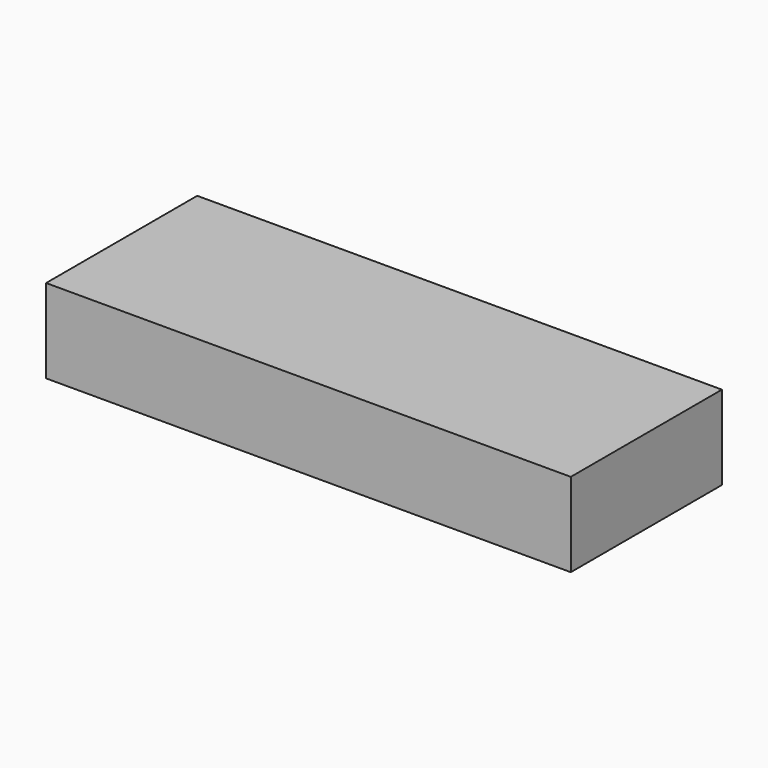
from build123d import *

# Parameters (mm, degrees)
F0_W     = 25
F0_H     = 9
F1_DEPTH = 4


# Not quite as in the source:
# - the program builds the solid bodies; features that only make, move or delete a surface that nothing else refers to are left out


with BuildPart() as f1:
    # F0 (on Top) → F1 (new body)
    with BuildSketch(Plane.XY):
        with Locations((-1.3542789966, -4.4008190995)):
            Rectangle(F0_W, F0_H)
    extrude(amount=F1_DEPTH)


solid = f1.part
